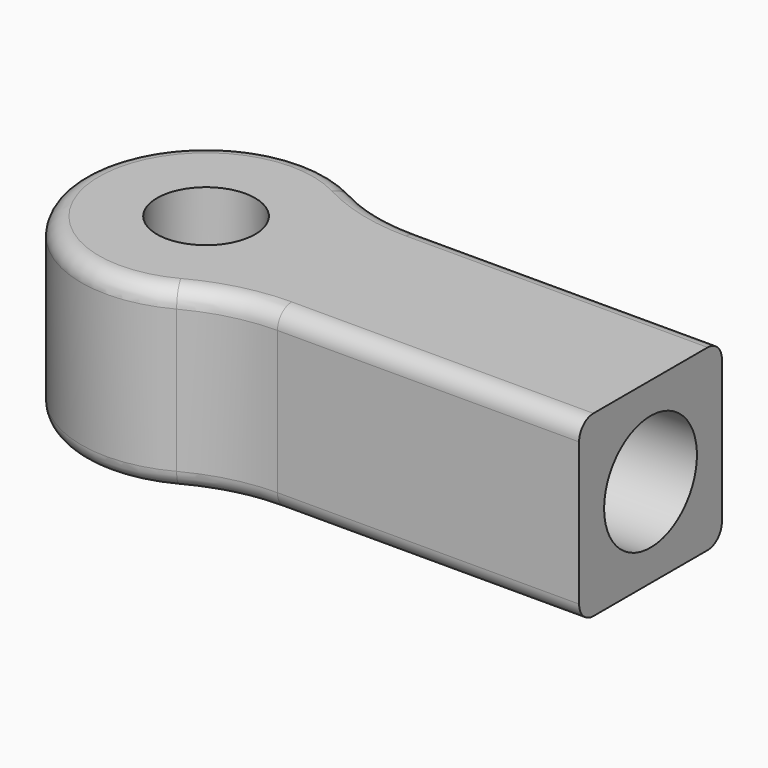
from build123d import *

# Parameters (mm, degrees)
F0_R     = 2.75
F1_DEPTH = 10
F2_R     = 10
F3_R     = 1
F5_D     = 6.5
F5_DEPTH = 15
F5_TIP   = 1.9527970118


# Not quite as in the source:
# - a feature names something its author has since deleted; it is built from what else it names


with BuildPart() as f1:
    # F0 (on Top) → F1 (new body)
    with BuildSketch(Plane.XY):
        with BuildLine():
            ThreePointArc((-2.9769337647, -5), (-1.4225088619, -2.7117470016), (-0.8759132502, 0))
            ThreePointArc((-0.8759132502, 0), (-1.4225088619, 2.7117470016), (-2.9769337647, 5))
            ThreePointArc((-2.9769337647, 5), (-14.8759132502, 0), (-2.9769337647, -5))
        make_face()
        with Locations((-7.8759132502, 0)):
            Circle(F0_R, mode=Mode.SUBTRACT)
        with BuildLine():
            ThreePointArc((-2.9769337647, 5), (-1.4225088619, 2.7117470016), (-0.8759132502, 0))
            ThreePointArc((-0.8759132502, 0), (-1.4225088619, -2.7117470016), (-2.9769337647, -5))
            Line((-2.9769337647, -5), (17.0230662353, -5))
            Line((17.0230662353, -5), (17.0230662353, 5))
            Line((17.0230662353, 5), (-2.9769337647, 5))
        make_face()
    extrude(amount=F1_DEPTH)

    # F2
    f2_edges = [f1.edges().sort_by_distance(p)[0] for p in [
        (-2.976934, 5, 5),
        (-2.976934, -5, 5),
    ]]
    fillet(f2_edges, radius=F2_R)

    # F3
    f3_edges = [f1.edges().sort_by_distance(p)[0] for p in [
        (8.573576, 5, 10),
        (-2.30127, 5.298575, 10),
        (8.573576, 5, 0),
    ]]
    fillet(f3_edges, radius=F3_R)

    # F5
    with Locations(Plane.YZ.offset(17.0230662353)):
        with Locations((0, 5)):
            Hole(F5_D / 2, depth=F5_DEPTH)
            with Locations((0, 0, -(F5_DEPTH + F5_TIP / 2))):  # 118° drill point
                Cone(0, F5_D / 2, F5_TIP, mode=Mode.SUBTRACT)


solid = f1.part
